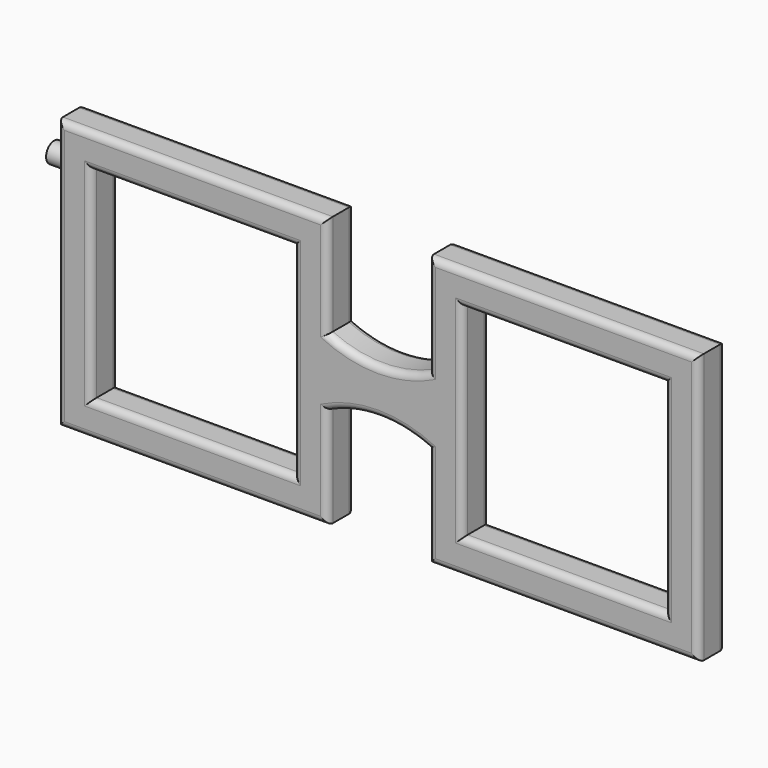
from build123d import *

# Parameters (mm, degrees)
F0_W     = 38.1
F0_H     = 38.1
F1_DEPTH = 6.35
F4_DEPTH = 6.35
F5_DEPTH = 6.351
F2_R     = 1.905
F6_DEPTH = 3.175
F7_R     = 1.26999


# Not quite as in the source:
# - a fillet or chamfer is up to 0.001 mm smaller than in the source, because OpenCascade refuses the exact size
# - a feature names something its author has since deleted; it is built from what else it names


with BuildPart() as f1:
    # F0 (on Front) → F1 (new body)
    with BuildSketch(Plane.XZ):
        Polygon((0, 12.7), (0, 31.75), (-50.8, 31.75), (-50.8, -19.05), (0, -19.05), (0, 0), (19.05, 0), (19.05, -19.05), (69.85, -19.05), (69.85, 31.75), (19.05, 31.75), (19.05, 12.7), align=None)
        with Locations((-25.4, 6.35)):
            Rectangle(F0_W, F0_H, mode=Mode.SUBTRACT)
        with Locations((44.45, 6.35)):
            Rectangle(F0_W, F0_H, mode=Mode.SUBTRACT)
    extrude(amount=F1_DEPTH)

    # F3 (on face) → F4 (join)
    with BuildSketch(Plane.XZ.offset(6.35)):
        with BuildLine():
            Line((0, 0), (19.05, 0))
            ThreePointArc((19.05, 0), (9.525, 2.0789034216), (0, 0))
        make_face()
        with BuildLine():
            Line((19.05, 12.7), (0, 12.7))
            ThreePointArc((0, 12.7), (9.525, 10.6210965784), (19.05, 12.7))
        make_face()
    extrude(amount=-F4_DEPTH)

    # F3 (on face) → F5 (cut, through all)
    with BuildSketch(Plane.XZ.offset(6.35)):
        with BuildLine():
            Line((0, 0), (19.05, 0))
            ThreePointArc((19.05, 0), (9.525, 2.0789034216), (0, 0))
        make_face()
        with BuildLine():
            Line((19.05, 12.7), (0, 12.7))
            ThreePointArc((0, 12.7), (9.525, 10.6210965784), (19.05, 12.7))
        make_face()
    extrude(amount=-F5_DEPTH, mode=Mode.SUBTRACT)

    # F2 (on face) → F6 (join, symmetric)
    with BuildSketch(Plane(origin=(-50.8, 0, 0), x_dir=(0, -1, 0), z_dir=(-1, 0, 0))):
        with Locations((3.175, 24.13)):
            Circle(F2_R)
    extrude(amount=F6_DEPTH, both=True)

    # F7 (radius 1.27 in the source; OpenCascade refuses exactly that, so slightly less here)
    f7_edges = [f1.edges().sort_by_distance(p)[0] for p in [
        (-25.4, -6.35, 31.75),
        (-50.8, -6.35, 6.35),
        (-25.4, -6.35, -19.05),
        (0, -6.35, -9.525),
        (0, -6.35, 22.225),
        (19.05, -6.35, 22.225),
        (19.05, -6.35, -9.525),
        (44.45, -6.35, -19.05),
        (69.85, -6.35, 6.35),
        (44.45, -6.35, 31.75),
        (44.45, 0, 31.75),
        (19.05, 0, 22.225),
        (0, 0, 22.225),
        (-25.4, 0, 31.75),
        (-50.8, 0, 6.35),
        (-25.4, 0, -19.05),
        (0, 0, -9.525),
        (19.05, 0, -9.525),
        (44.45, 0, -19.05),
        (69.85, 0, 6.35),
        (9.525, -6.35, 10.621097),
        (9.525, 0, 10.621097),
        (9.525, 0, 2.078903),
        (9.525, -6.35, 2.078903),
        (25.4, -6.35, 6.35),
        (25.4, 0, 6.35),
        (44.45, -6.35, -12.7),
        (44.45, 0, -12.7),
        (63.5, -6.35, 6.35),
        (63.5, 0, 6.35),
        (44.45, 0, 25.4),
        (44.45, -6.35, 25.4),
        (-25.4, -6.35, 25.4),
        (-25.4, 0, 25.4),
        (-44.45, 0, 6.35),
        (-44.45, -6.35, 6.35),
        (-25.4, 0, -12.7),
        (-25.4, -6.35, -12.7),
        (-6.35, 0, 6.35),
        (-6.35, -6.35, 6.35),
    ]]
    fillet(f7_edges, radius=F7_R)


solid = f1.part
